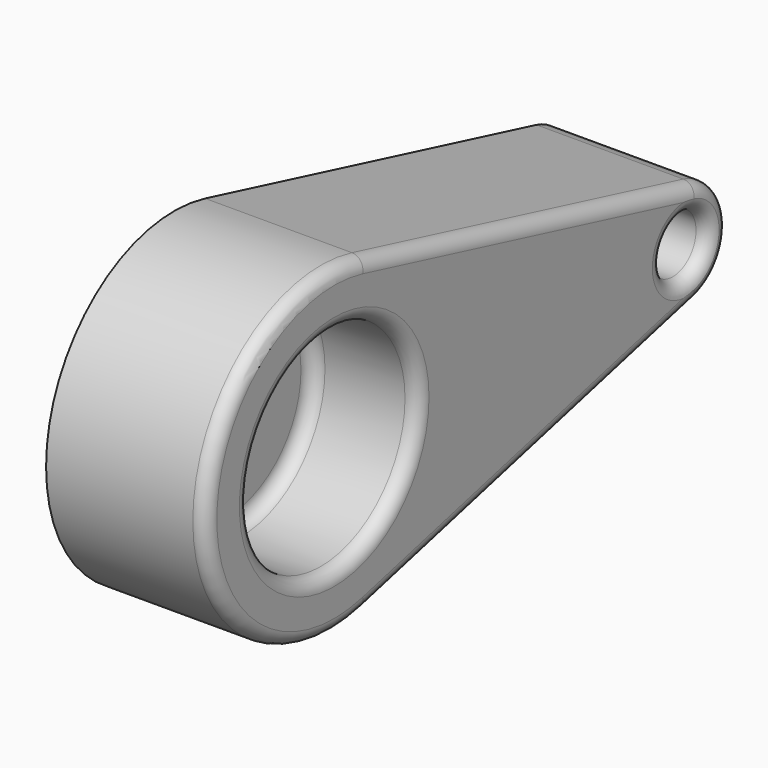
from build123d import *

# Parameters (mm, degrees)
F1_DEPTH     = 76.2
F2_R         = 50.0828504331
F2_R_2       = 13.7976444657
F3_DEPTH     = 50.8
F4_T         = -2.54
F5_T3_DEPTH  = 203.2
F5_T5_DEPTH  = 203.2
F5_T8_ANGLE  = 208.0724869359
F5_T10_ANGLE = 151.9275130641


# Not quite as in the source:
# - a fillet or chamfer that OpenCascade refuses, or shapes differently, is made with other operations: its cross-section is extruded or revolved along the edge and cut away or added


with BuildPart() as f1:
    # F0 (on Right) → F1 (new body)
    with BuildSketch(Plane.YZ):
        with BuildLine():
            ThreePointArc((18.4812146278, -73.9248585111), (60.0612543768, -46.8944103565), (76.2, 0))
            ThreePointArc((76.2, 0), (60.0612543768, 46.8944103565), (18.4812146278, 73.9248585111))
            ThreePointArc((18.4812146278, 73.9248585111), (-76.2, 0), (18.4812146278, -73.9248585111))
        make_face()
        with BuildLine():
            ThreePointArc((18.4812146278, 73.9248585111), (60.0612543768, 46.8944103565), (76.2, 0))
            ThreePointArc((76.2, 0), (60.0612543768, -46.8944103565), (18.4812146278, -73.9248585111))
            Line((18.4812146278, -73.9248585111), (215.6141706573, -24.6416195037))
            ThreePointArc((215.6141706573, -24.6416195037), (184.0537657814, 0), (215.6141706573, 24.6416195037))
            Line((215.6141706573, 24.6416195037), (18.4812146278, 73.9248585111))
        make_face()
        with BuildLine():
            ThreePointArc((234.8537657814, 0), (229.474183907, 15.6314701188), (215.6141706573, 24.6416195037))
            ThreePointArc((215.6141706573, 24.6416195037), (184.0537657814, 0), (215.6141706573, -24.6416195037))
            ThreePointArc((215.6141706573, -24.6416195037), (229.474183907, -15.6314701188), (234.8537657814, 0))
        make_face()
    extrude(amount=F1_DEPTH)

    # F2 (on face) → F3 (cut)
    with BuildSketch(Plane.YZ.offset(76.2)):
        Circle(F2_R)
        with Locations((209.4537657814, 0)):
            Circle(F2_R_2)
    extrude(amount=-F3_DEPTH, mode=Mode.SUBTRACT)

    # F4
    f4_openings = [f1.faces().sort_by_distance(p)[0] for p in [
        (0, 57.51924, 0),
    ]]
    offset(amount=F4_T, openings=f4_openings, kind=Kind.INTERSECTION)

    # F5: fillet of radius 6.35 on 7 edges, made by hand

    # F5_s1 → F5_t2 (revolve)
    with BuildSketch(Plane.XY):
        with BuildLine():
            ThreePointArc((31.75, 50.0828504331), (27.2598719395, 48.2229784936), (25.4, 43.7328504331))
            Line((25.4, 43.7328504331), (25.4, 50.0828504331))
            Line((25.4, 50.0828504331), (31.75, 50.0828504331))
        make_face()
    revolve(axis=Axis((25.4, 0, 0), (1, 0, 0)))

    # F5_s4 → F5_t3 (cut)
    with BuildSketch(Plane(origin=(0, 197.1329560295, -49.2832390074), x_dir=(1, 0, 0), z_dir=(0, -0.9701425001, 0.242535625))):
        with BuildLine():
            ThreePointArc((69.85, 76.2), (74.3401280605, 74.3401280605), (76.2, 69.85))
            Line((76.2, 69.85), (76.2, 76.2))
            Line((76.2, 76.2), (69.85, 76.2))
        make_face()
    extrude(amount=F5_T3_DEPTH, mode=Mode.SUBTRACT)

    # F5_s6 → F5_t5 (cut)
    with BuildSketch(Plane(origin=(0, 0, 0), x_dir=(1, 0, 0), z_dir=(0, 0.9701425001, 0.242535625))):
        with BuildLine():
            ThreePointArc((69.85, 76.2), (74.3401280605, 74.3401280605), (76.2, 69.85))
            Line((76.2, 69.85), (76.2, 76.2))
            Line((76.2, 76.2), (69.85, 76.2))
        make_face()
    extrude(amount=F5_T5_DEPTH, mode=Mode.SUBTRACT)

    # F5_s7 → F5_t8 (revolve, cut)
    with BuildSketch(Plane(origin=(0, 0, 0), x_dir=(1, 0, 0), z_dir=(0, 0.9701425001, -0.242535625))):
        with BuildLine():
            ThreePointArc((69.85, -76.2), (74.3401280605, -74.3401280605), (76.2, -69.85))
            Line((76.2, -69.85), (76.2, -76.2))
            Line((76.2, -76.2), (69.85, -76.2))
        make_face()
    revolve(axis=Axis((76.2, 0, 0), (1, 0, 0)), revolution_arc=F5_T8_ANGLE, mode=Mode.SUBTRACT)

    # F5_s9 → F5_t10 (revolve, cut)
    with BuildSketch(Plane(origin=(0, 197.1329560295, 49.2832390074), x_dir=(1, 0, 0), z_dir=(0, -0.9701425001, -0.242535625))):
        with BuildLine():
            ThreePointArc((76.2, -69.85), (74.3401280605, -74.3401280605), (69.85, -76.2))
            Line((69.85, -76.2), (76.2, -76.2))
            Line((76.2, -76.2), (76.2, -69.85))
        make_face()
    revolve(axis=Axis((76.2, 209.4537657814, 0), (1, 0, 0)), revolution_arc=F5_T10_ANGLE, mode=Mode.SUBTRACT)

    # F5_s11 → F5_t12 (revolve, cut)
    with BuildSketch(Plane.XY):
        with BuildLine():
            ThreePointArc((76.2, 56.4328504331), (74.3401280605, 51.9427223726), (69.85, 50.0828504331))
            Line((69.85, 50.0828504331), (76.2, 50.0828504331))
            Line((76.2, 50.0828504331), (76.2, 56.4328504331))
        make_face()
    revolve(axis=Axis((76.2, 0, 0), (1, 0, 0)), mode=Mode.SUBTRACT)

    # F5_s13 → F5_t14 (revolve, cut)
    with BuildSketch(Plane.XY):
        with BuildLine():
            ThreePointArc((76.2, 229.6014102471), (74.3401280605, 225.1112821866), (69.85, 223.2514102471))
            Line((69.85, 223.2514102471), (76.2, 223.2514102471))
            Line((76.2, 223.2514102471), (76.2, 229.6014102471))
        make_face()
    revolve(axis=Axis((76.2, 209.4537657814, 0), (1, 0, 0)), mode=Mode.SUBTRACT)


solid = f1.part
